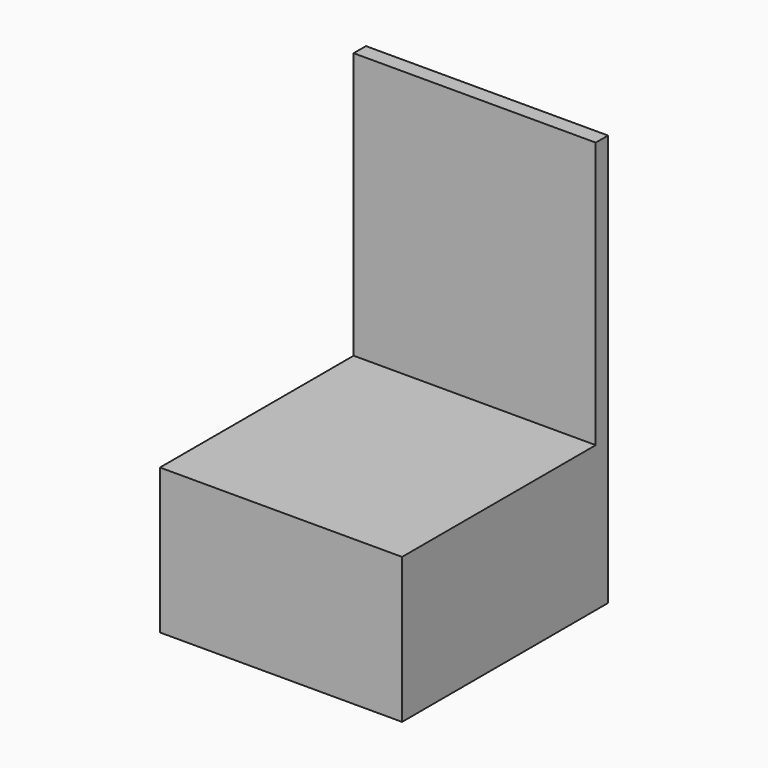
from build123d import *

# Parameters (mm, degrees)
F0_W     = 50
F0_H     = 50
F1_DEPTH = 30
F2_W     = 50
F2_H     = 30
F2_H_2   = 55
F3_DEPTH = 3.175
F4_R     = 5


# Not quite as in the source:
# - an extrude whose draft closes it to a point is written as a loft to that point


with BuildPart() as f1:
    # F0 (on Top) → F1 (new body)
    with BuildSketch(Plane.XY):
        with Locations((-20.7551017412, -14.590555802)):
            Rectangle(F0_W, F0_H)
    extrude(amount=F1_DEPTH)

    # F2 (on face) → F3 (join)
    with BuildSketch(Plane(origin=(0, 10.409444198, 0), x_dir=(-1, 0, 0), z_dir=(0, 1, 0))):
        with Locations((20.7551017412, 15)):
            Rectangle(F2_W, F2_H)
        with Locations((20.7551017412, 57.5)):
            Rectangle(F2_W, F2_H_2)
    extrude(amount=F3_DEPTH)

    # F4 (on face) → F5 section 0
    with BuildSketch(Plane(origin=(0, 0, 0), x_dir=(1, 0, 0), z_dir=(0, 0, -1)), mode=Mode.PRIVATE) as f5_s0:
        with Locations((-20.7551017412, 14.5431621725)):
            Circle(F4_R)
    loft([f5_s0.sketch, Vertex(-20.7551017412, -14.5431621725, -5.958767963)], ruled=True)


solid = f1.part
